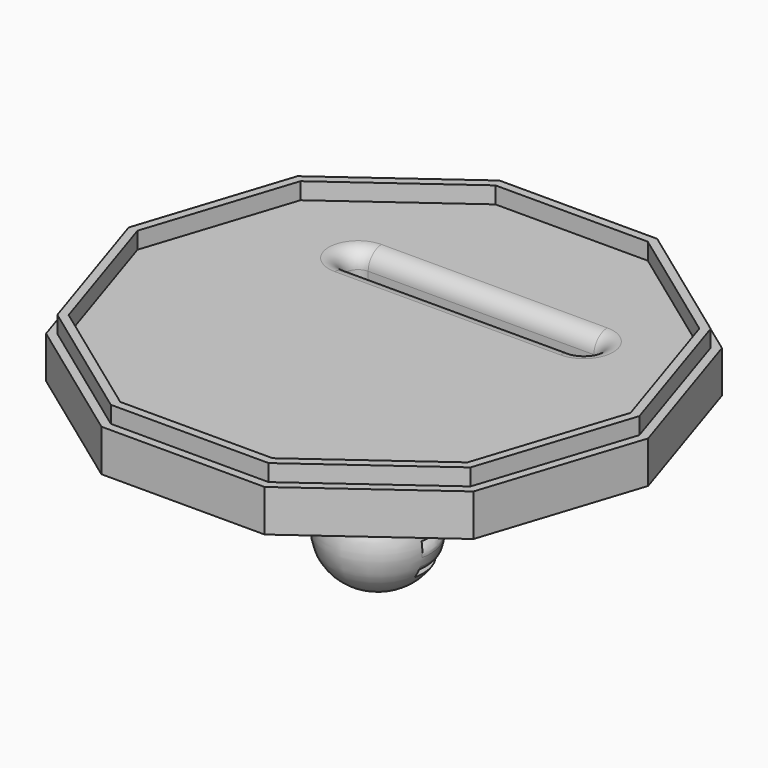
from build123d import *

# Parameters (mm, degrees)
F1_DEPTH     = 6.35
F3_DEPTH     = 2.54
F4_TEXT_SIZE = 14.7994349702
F5_DEPTH     = 2.54
F8_R         = 2.54
F9_R         = 0.635
F12_DEPTH    = 7.62
F13_R        = 1.27


# Not quite as in the source:
# - Text() gives the source's letters only with a copy of the font that has no kerning and outlines rounded to 1/6400 em; it was checked with that copy


with BuildPart() as f1:
    # F0 (on Top) → F1 (new body)
    with BuildSketch(Plane.XY):
        Polygon((12.3794404265, 38.1), (-12.3794404265, 38.1), (-32.4097957982, 23.5470949714), (-40.0607107435, 0), (-32.4097957982, -23.5470949714), (-12.3794404265, -38.1), (12.3794404265, -38.1), (32.4097957982, -23.5470949714), (40.0607107435, 0), (32.4097957982, 23.5470949714), align=None)
        with BuildLine():
            Line((18.5746420175, 12.7584074706), (-15.654521063, 12.7584074706))
            ThreePointArc((-15.654521063, 12.7584074706), (-17.559521063, 14.6634074706), (-15.654521063, 16.5684074706))
            Line((-15.654521063, 16.5684074706), (18.5746420175, 16.5684074706))
            ThreePointArc((18.5746420175, 16.5684074706), (20.4796420175, 14.6634074706), (18.5746420175, 12.7584074706))
        make_face(mode=Mode.SUBTRACT)
    extrude(amount=F1_DEPTH)

    # F2 (on face) → F3 (join)
    with BuildSketch(Plane.XY.offset(6.35)):
        Polygon((-11.9667924123, 36.83), (-31.3294692716, 22.7621918057), (-38.7253537187, 0), (-31.3294692716, -22.7621918057), (-11.9667924123, -36.83), (11.9667924123, -36.83), (31.3294692716, -22.7621918057), (38.7253537187, 0), (31.3294692716, 22.7621918057), (11.9667924123, 36.83), align=None)
        Polygon((-30.249142745, 21.9772886399), (-11.554144398, 35.56), (11.554144398, 35.56), (30.249142745, 21.9772886399), (37.3899966939, 0), (30.249142745, -21.9772886399), (11.554144398, -35.56), (-11.554144398, -35.56), (-30.249142745, -21.9772886399), (-37.3899966939, 0), align=None, mode=Mode.SUBTRACT)
    extrude(amount=F3_DEPTH)

    # F4 (on face) → F5 (cut)
    with BuildSketch(Plane(origin=(0, 0, 0), x_dir=(1, 0, 0), z_dir=(0, 0, -1))):
        with Locations((-33.9275897478, 7.6530016443)):
            Text("Josh's bin", F4_TEXT_SIZE, font='Open Sans', text_align=(TextAlign.LEFT, TextAlign.BOTTOM))
    extrude(amount=-F5_DEPTH, mode=Mode.SUBTRACT)

    # F8
    f8_edges = [f1.edges().sort_by_distance(p)[0] for p in [
        (-17.559521, 14.663407, 0),
        (1.46006, 12.758407, 6.35),
        (20.479642, 14.663407, 6.35),
        (1.46006, 16.568407, 6.35),
        (-17.559521, 14.663407, 6.35),
    ]]
    fillet(f8_edges, radius=F8_R)


with BuildPart() as f7:
    # F6 (on Right) → F7 (revolve)
    with BuildSketch(Plane.YZ):
        with BuildLine():
            Line((-1.1781250865, 0), (-2.4798750865, 0))
            Line((-2.4798750865, 0), (-2.4798750865, -10.8318541475))
            ThreePointArc((-2.4798750865, -10.8318541475), (-9.1118030127, -18.7680720737), (-1.1755850865, -25.4))
            Line((-1.1755850865, -25.4), (-1.1755850865, -23.5402363628))
            Line((-1.1755850865, -23.5402363628), (-1.2392633704, -12.2314024928))
            Line((-1.2392633704, -12.2314024928), (-1.1781250865, 0))
        make_face()
    revolve(axis=Axis((0, -1.1755850865, -12.7), (0, 0, -1)))

    # F9
    f9_edges = [f7.edges().sort_by_distance(p)[0] for p in [
        (0, 0.128705, -10.831854),
    ]]
    fillet(f9_edges, radius=F9_R)

    # F11 (on offset) → F12 (cut)
    with BuildSketch(Plane(origin=(0, 5.08, 0), x_dir=(-1, 0, 0), z_dir=(0, 1, 0))):
        Polygon((-12.4940212602, -22.0186752397), (12.9059787398, -22.0186752397), (12.8521079608, -21.2585818644), (-12.5478920392, -21.2585818644), align=None)
        Polygon((-12.5771392103, -17.6177665738), (12.8228607897, -17.6177665738), (12.7689900107, -16.8576731985), (-12.6310099893, -16.8576731985), align=None)
    extrude(amount=-F12_DEPTH, mode=Mode.SUBTRACT)

    # F13
    f13_edges = [f7.edges().sort_by_distance(p)[0] for p in [
        (-6.609685, 1.817242, -21.258582),
        (6.609685, 1.817242, -21.258582),
        (-7.419836, 1.674427, -17.617767),
        (7.419836, 1.674427, -17.617767),
    ]]
    fillet(f13_edges, radius=F13_R)


solid = Compound([f1.part, f7.part])
